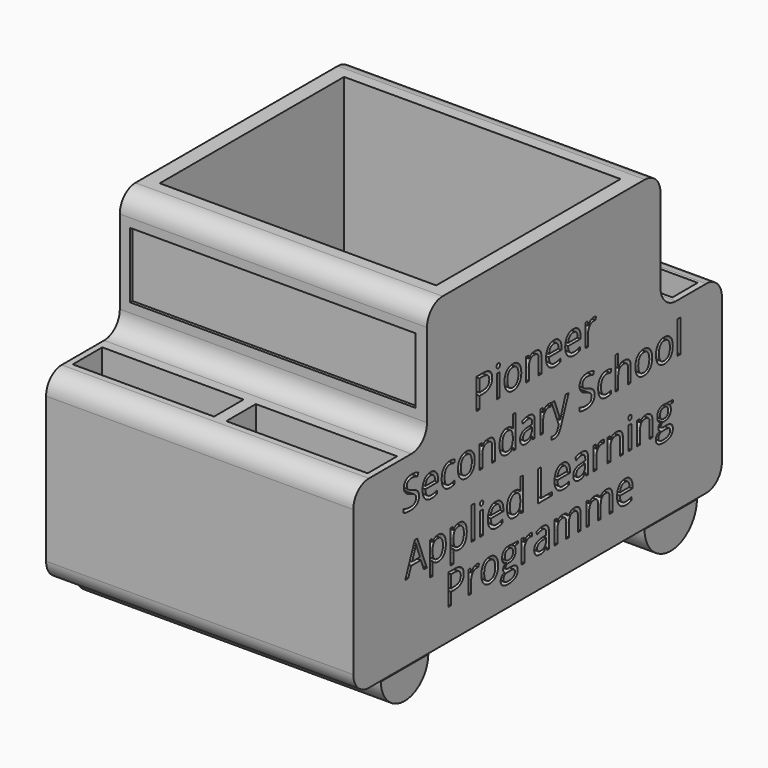
from build123d import *

# Parameters (mm, degrees)
F1_DEPTH     = 50
F2_W         = 90
F2_H         = 75
F3_DEPTH     = 95
F4_W         = 46
F4_H         = 12
F5_DEPTH     = 55
F6_W         = 96
F6_H         = 10.3
F7_DEPTH     = 55
F8_TEXT_SIZE = 13.8888888889
F9_DEPTH     = 25
F11_DEPTH    = 50
F12_W        = 92.9185636342
F12_H        = 21.3769711554
F13_DEPTH    = 1


# Not quite as in the source:
# - Text() gives the source's letters only with a copy of the font that has no kerning and outlines rounded to 1/6400 em; it was checked with that copy


with BuildPart() as f1:
    # F0 (on Right) → F1 (new body, symmetric)
    with BuildSketch(Plane.YZ):
        with BuildLine():
            Line((-51.35, 40), (-68.65, 40))
            ThreePointArc((-68.65, 40), (-73.1401280605, 38.1401280605), (-75, 33.65))
            Line((-75, 33.65), (-75, -13.65))
            ThreePointArc((-75, -13.65), (-73.1401280605, -18.1401280605), (-68.65, -20))
            Line((-68.65, -20), (68.65, -20))
            ThreePointArc((68.65, -20), (73.1401280605, -18.1401280605), (75, -13.65))
            Line((75, -13.65), (75, 33.65))
            ThreePointArc((75, 33.65), (73.1401280605, 38.1401280605), (68.65, 40))
            Line((68.65, 40), (56.35, 40))
            ThreePointArc((56.35, 40), (51.8598719395, 41.8598719395), (50, 46.35))
            Line((50, 46.35), (50, 73.65))
            ThreePointArc((50, 73.65), (48.1401280605, 78.1401280605), (43.65, 80))
            Line((43.65, 80), (-38.65, 80))
            ThreePointArc((-38.65, 80), (-43.1401280605, 78.1401280605), (-45, 73.65))
            Line((-45, 73.65), (-45, 46.35))
            ThreePointArc((-45, 46.35), (-46.8598719395, 41.8598719395), (-51.35, 40))
        make_face()
    extrude(amount=F1_DEPTH, both=True)

    # F2 (on face) → F3 (cut)
    with BuildSketch(Plane.XY.offset(80)):
        with Locations((0, 2.5)):
            Rectangle(F2_W, F2_H)
    extrude(amount=-F3_DEPTH, mode=Mode.SUBTRACT)

    # F4 (on face) → F5 (cut)
    with BuildSketch(Plane.XY.offset(40)):
        with Locations((-25, -60.65)):
            Rectangle(F4_W, F4_H)
        with Locations((25, -60.65)):
            Rectangle(F4_W, F4_H)
    extrude(amount=-F5_DEPTH, mode=Mode.SUBTRACT)

    # F6 (on face) → F7 (cut)
    with BuildSketch(Plane.XY.offset(40)):
        with Locations((0, 62.5)):
            Rectangle(F6_W, F6_H)
    extrude(amount=-F7_DEPTH, mode=Mode.SUBTRACT)

    # F8 (on face) → F9 (cut)
    with BuildSketch(Plane.YZ.offset(50)):
        with Locations((-26.1228942376, 41.4392124645)):
            Text('Pioneer', F8_TEXT_SIZE, font='Open Sans', text_align=(TextAlign.LEFT, TextAlign.BOTTOM))
        with Locations((-55.2165061235, 24.0465866029)):
            Text('Secondary School', F8_TEXT_SIZE, font='Open Sans', text_align=(TextAlign.LEFT, TextAlign.BOTTOM))
        with Locations((-53.8591481745, 4.8174185306)):
            Text('Applied Learning', F8_TEXT_SIZE, font='Open Sans', text_align=(TextAlign.LEFT, TextAlign.BOTTOM))
        with Locations((-37.7112010099, -10)):
            Text('Programme', F8_TEXT_SIZE, font='Open Sans', text_align=(TextAlign.LEFT, TextAlign.BOTTOM))
    extrude(amount=-F9_DEPTH, mode=Mode.SUBTRACT)

    # F12 (on face) → F13 (cut)
    with BuildSketch(Plane.XZ.offset(45)):
        with Locations((-0.2850275487, 60.0753035396)):
            Rectangle(F12_W, F12_H)
    extrude(amount=-F13_DEPTH, mode=Mode.SUBTRACT)


with BuildPart() as f11:
    # F10 (on Right) → F11 (new body, symmetric)
    with BuildSketch(Plane.YZ):
        with BuildLine():
            Line((-44.4678603171, -20.2182786635), (-63.7883618474, -20.2211998403))
            ThreePointArc((-63.7883618474, -20.2211998403), (-54.1266756765, -29.7134332788), (-44.4678603171, -20.2182786635))
        make_face()
    extrude(amount=F11_DEPTH, both=True)


with BuildPart() as f11b:
    # F10 (on Right) → F11, piece 2 (new body, symmetric)
    with BuildSketch(Plane.YZ):
        with BuildLine():
            ThreePointArc((43.4903603975, -20.1758814671), (54.1454139945, -30.7301342026), (64.8451671004, -20.2211998403))
            Line((64.8451671004, -20.2211998403), (43.4903603975, -20.1758814671))
        make_face()
    extrude(amount=F11_DEPTH, both=True)


solid = Compound([f1.part, f11.part, f11b.part])
